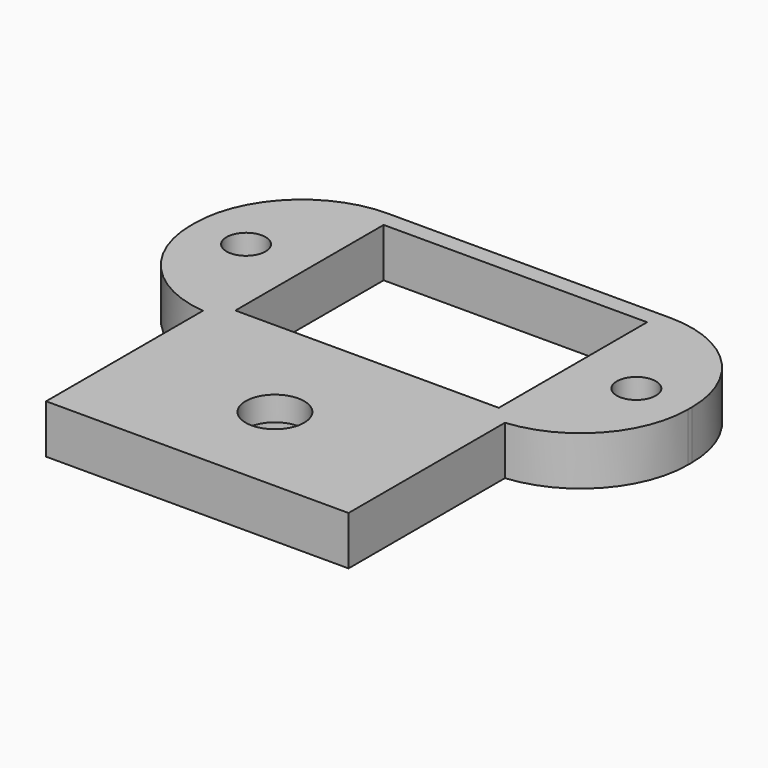
from build123d import *

# Parameters (mm, degrees)
F0_W         = 31
F0_H         = 22.5
F0_W_2       = 27
F0_H_2       = 19
F1_DEPTH     = 5
F2_DEPTH     = 20
F3_W         = 22.4636928365
F3_H         = 5
F4_DEPTH     = 10
F5_W         = 22.3973267898
F5_H         = 5
F6_DEPTH     = 10
F7_R         = 3
F7_R_2       = 2
F8_DEPTH     = 25
F7_R_3       = 5
F9_DEPTH     = 2.5
F10_T1_DEPTH = 59.7722557505
F10_T3_DEPTH = 60


# Not quite as in the source:
# - a fillet or chamfer that OpenCascade refuses, or shapes differently, is made with other operations: its cross-section is extruded or revolved along the edge and cut away or added


with BuildPart() as f1:
    # F0 (on Top) → F1 (new body)
    with BuildSketch(Plane.XY):
        Rectangle(F0_W, F0_H)
        Rectangle(F0_W_2, F0_H_2, mode=Mode.SUBTRACT)
    extrude(amount=F1_DEPTH)

    # F2 (add): a face of the model
    f2_faces = [f1.faces().sort_by_distance(p)[0] for p in [
        (0, -11.25, 2.5),
    ]]
    extrude(f2_faces, amount=F2_DEPTH)

    # F3 (on face) → F4 (join)
    with BuildSketch(Plane.YZ.offset(15.5)):
        with Locations((0.0181535818, 2.5)):
            Rectangle(F3_W, F3_H)
    extrude(amount=F4_DEPTH)

    # F5 (on face) → F6 (join)
    with BuildSketch(Plane(origin=(-15.5, 0, 0), x_dir=(0, -1, 0), z_dir=(-1, 0, 0))):
        with Locations((-0.0513366051, 2.5)):
            Rectangle(F5_W, F5_H)
    extrude(amount=F6_DEPTH)

    # F7 (on face) → F8 (cut)
    with BuildSketch(Plane(origin=(0, 0, 0), x_dir=(1, 0, 0), z_dir=(0, 0, -1))):
        with Locations((-0.0447025523, 21.25)):
            Circle(F7_R)
        with Locations((20, 0)):
            Circle(F7_R_2)
        with Locations((-20, 0)):
            Circle(F7_R_2)
    extrude(amount=-F8_DEPTH, mode=Mode.SUBTRACT)

    # F7 (on face) → F9 (cut)
    with BuildSketch(Plane(origin=(0, 0, 0), x_dir=(1, 0, 0), z_dir=(0, 0, -1))):
        with Locations((-0.0447025523, 21.25)):
            Circle(F7_R_3)
        with Locations((-0.0447025523, 21.25)):
            Circle(F7_R, mode=Mode.SUBTRACT)
        Polygon((21.7320508076, 3), (18.2679491924, 3), (16.5358983849, 0), (18.2679491924, -3), (21.7320508076, -3), (23.4641016151, 0), align=None)
        with Locations((20, 0)):
            Circle(F7_R_2, mode=Mode.SUBTRACT)
        Polygon((-18.2679491924, 3), (-21.7320508076, 3), (-23.4641016151, 0), (-21.7320508076, -3), (-18.2679491924, -3), (-16.5358983849, 0), align=None)
        with Locations((-20, 0)):
            Circle(F7_R_2, mode=Mode.SUBTRACT)
    extrude(amount=-F9_DEPTH, mode=Mode.SUBTRACT)

    # F10: fillet of radius 11 on 7 edges, made by hand

    # F10_s2 → F10_t1 (cut)
    with BuildSketch(Plane.XY.offset(-27.3861278753)):
        with BuildLine():
            ThreePointArc((-15.5, -11.1473267898), (-22.6240384046, -7.6090741268), (-25.5, -0.1928756397))
            Line((-25.5, -0.1928756397), (-25.5, -11.1473267898))
            Line((-25.5, -11.1473267898), (-15.5, -11.1473267898))
        make_face()
        with BuildLine():
            ThreePointArc((15.5, -11.2136928365), (22.6240384046, -7.6754401735), (25.5, -0.2592416864))
            Line((25.5, -0.2592416864), (25.5, -11.2136928365))
            Line((25.5, -11.2136928365), (15.5, -11.2136928365))
        make_face()
    extrude(amount=F10_T1_DEPTH, mode=Mode.SUBTRACT)

    # F10_s4 → F10_t3 (cut)
    with BuildSketch(Plane.XY.offset(-27.5)):
        with BuildLine():
            ThreePointArc((25.5, 0.25), (22.2781745931, 8.0281745931), (14.5, 11.25))
            Line((14.5, 11.25), (25.5, 11.25))
            Line((25.5, 11.25), (25.5, 0.25))
        make_face()
        with BuildLine():
            ThreePointArc((-14.5, 11.25), (-22.2781745931, 8.0281745931), (-25.5, 0.25))
            Line((-25.5, 0.25), (-25.5, 11.25))
            Line((-25.5, 11.25), (-14.5, 11.25))
        make_face()
    extrude(amount=F10_T3_DEPTH, mode=Mode.SUBTRACT)


solid = f1.part
